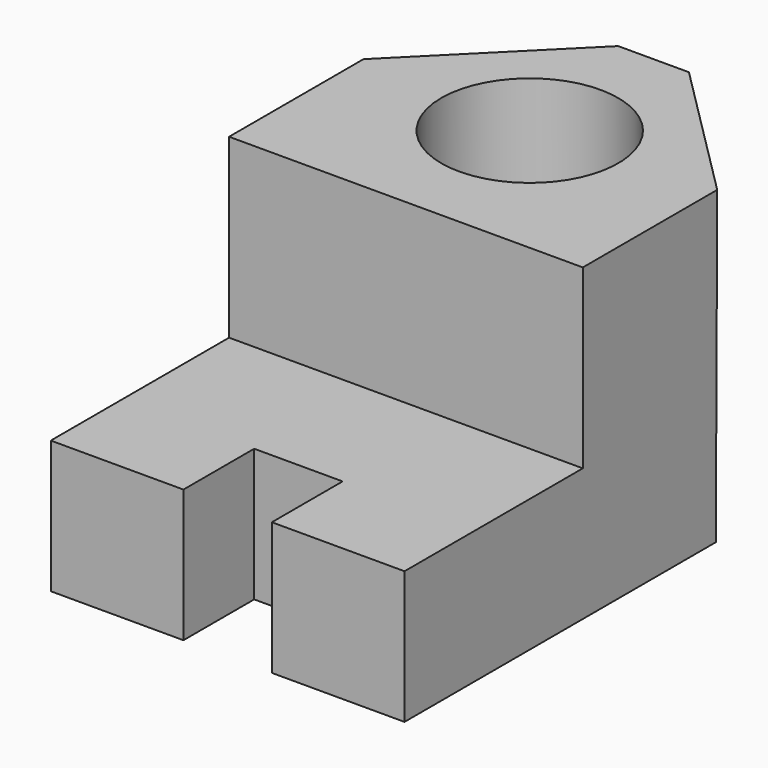
from build123d import *

# Parameters (mm, degrees)
F1_DEPTH = 50.8
F3_D     = 25.4
F4_SIZE  = 20.32
F5_W     = 12.7
F5_H     = 12.7
F6_DEPTH = 0.254
F7_DEPTH = 35.052


with BuildPart() as f1:
    # F0 (on Right) → F1 (new body)
    with BuildSketch(Plane.YZ):
        Polygon((-24.5744947175, 0), (-40.5764947175, 0), (-40.5764947175, -19.05), (35.6235052825, -19.05), (35.8775052825, 25.4), (-8.5724947175, 25.4), (-8.5724947175, 0), align=None)
    extrude(amount=F1_DEPTH)

    # F3 (through all)
    with Locations(Plane.XY.offset(25.4)):
        with Locations((25.4, 13.6525052825)):
            Hole(F3_D / 2)

    # F4
    f4_edges = [f1.edges().sort_by_distance(p)[0] for p in [
        (0, 35.750505, 3.175),
        (50.8, 35.750505, 3.175),
    ]]
    chamfer(f4_edges, length=F4_SIZE)

    # F5 (on face) → F6 (join)
    with BuildSketch(Plane.XY):
        with Locations((25.4, -34.2264947175)):
            Rectangle(F5_W, F5_H)
    extrude(amount=F6_DEPTH)

    # F7 (cut): a face of the model
    f7_faces = [f1.faces().sort_by_distance(p)[0] for p in [
        (25.4, -34.2264947175, 0.254),
    ]]
    extrude(f7_faces, amount=-F7_DEPTH, mode=Mode.SUBTRACT)


solid = f1.part
